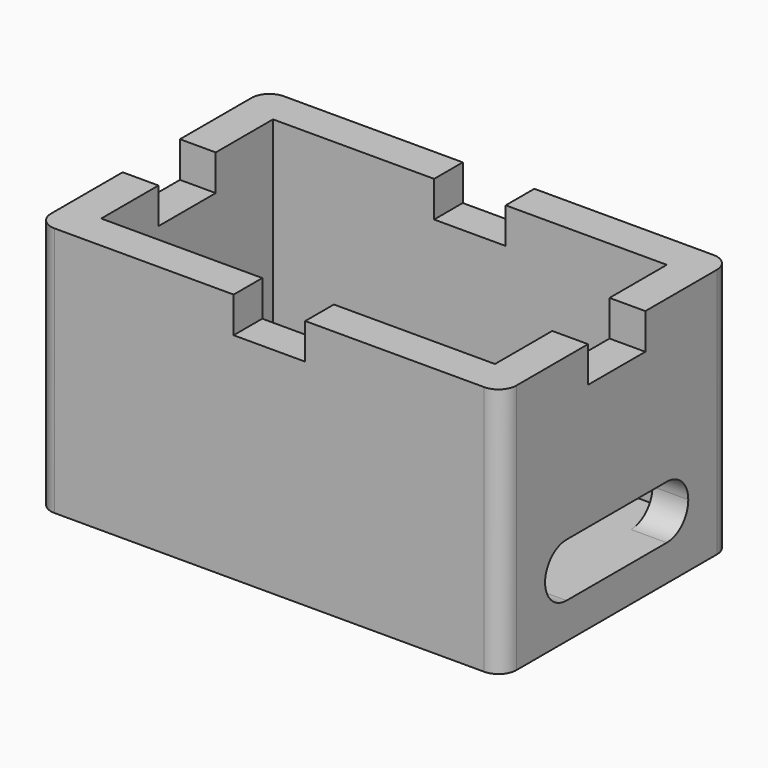
from build123d import *

# Parameters (mm, degrees)
F1_DEPTH = 10
F2_W     = 130
F2_H     = 80
F2_W_2   = 110
F2_H_2   = 60
F3_DEPTH = 60
F4_W     = 20
F4_H     = 10
F4_W_2   = 10
F4_H_2   = 20
F5_DEPTH = 10
F6_R     = 5
F8_DEPTH = 25
F9_R     = 7.49999


# Not quite as in the source:
# - a fillet or chamfer is up to 0.001 mm smaller than in the source, because OpenCascade refuses the exact size


with BuildPart() as f1:
    # F0 (on Top) → F1 (new body)
    with BuildSketch(Plane.XY):
        Polygon((55, 40), (-55, 40), (-65, 40), (-65, -40), (-55, -40), (65, -40), (65, -30), (65, 40), align=None)
    extrude(amount=F1_DEPTH)

    # F2 (on face) → F3 (join)
    with BuildSketch(Plane.XY.offset(10)):
        Rectangle(F2_W, F2_H)
        Rectangle(F2_W_2, F2_H_2, mode=Mode.SUBTRACT)
    extrude(amount=F3_DEPTH)

    # F4 (on face) → F5 (cut)
    with BuildSketch(Plane.XY.offset(70)):
        Polygon((10, 30), (10, 40), (0, 40), (-10, 40), (-10, 30), align=None)
        Polygon((-65, 0), (-65, -10), (-55, -10), (-55, 10), (-65, 10), align=None)
        with Locations((0, -35)):
            Rectangle(F4_W, F4_H)
        with Locations((60, 0)):
            Rectangle(F4_W_2, F4_H_2)
    extrude(amount=-F5_DEPTH, mode=Mode.SUBTRACT)

    # F6
    f6_edges = [f1.edges().sort_by_distance(p)[0] for p in [
        (-65, -40, 35),
        (65, -40, 35),
        (-65, 40, 35),
        (65, 40, 35),
    ]]
    fillet(f6_edges, radius=F6_R)

    # F7 (on face) → F8 (cut)
    with BuildSketch(Plane.YZ.offset(65)):
        Polygon((-25, 10), (0, 10), (25, 10), (25, 25), (-25, 25), align=None)
    extrude(amount=-F8_DEPTH, mode=Mode.SUBTRACT)

    # F9 (radius 7.5 in the source; OpenCascade refuses exactly that, so slightly less here)
    f9_edges = [f1.edges().sort_by_distance(p)[0] for p in [
        (60, 25, 25),
        (60, 25, 10),
        (60, -25, 10),
        (60, -25, 25),
    ]]
    fillet(f9_edges, radius=F9_R)


solid = f1.part
